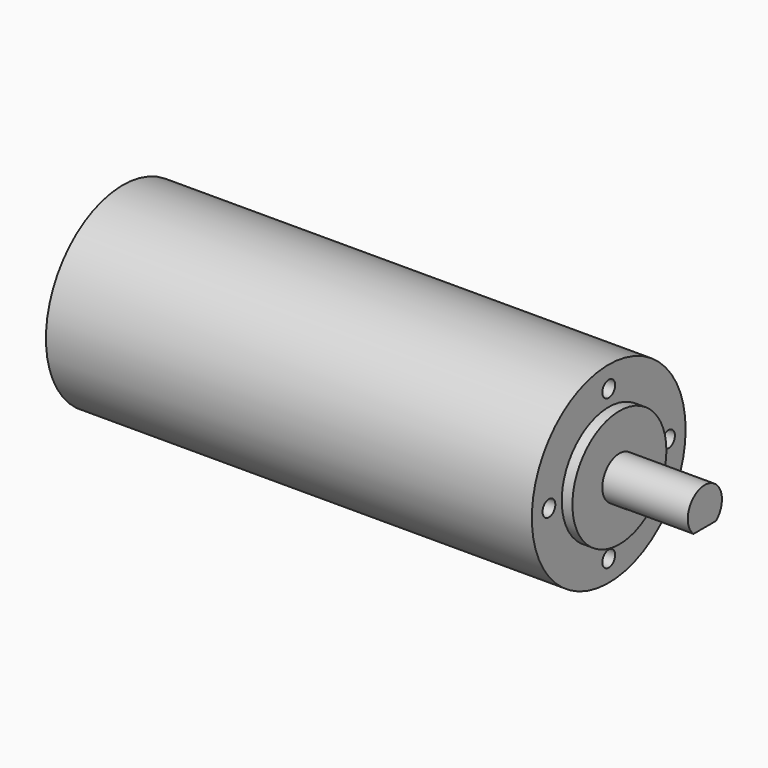
from build123d import *

# Parameters (mm, degrees)
F0_R            = 18
F1_DEPTH        = 91
F2_R            = 11
F3_DEPTH        = 2
F4_R            = 4
F5_DEPTH        = 18
F6_R            = 1.5
F7_DEPTH        = 5
F7_COPIES_COUNT = 4
F9_START        = 5
F8_W            = 20
F8_H            = 10
F9_DEPTH        = 20


# Not quite as in the source:
# - a pattern or mirror of a feature is missing from the dataset's text; its kind, count and spacing are read off the source's solid


with BuildPart() as f1:
    # F0 (on Right) → F1 (new body)
    with BuildSketch(Plane.YZ):
        Circle(F0_R)
    extrude(amount=-F1_DEPTH)

    # F2 (on Right) → F3 (join)
    with BuildSketch(Plane.YZ):
        Circle(F2_R)
    extrude(amount=F3_DEPTH)

    # F4 (on Right) → F5 (join)
    with BuildSketch(Plane.YZ):
        Circle(F4_R)
    extrude(amount=F5_DEPTH)

    # F6 (on Right) → F7 (cut)
    with BuildSketch(Plane.YZ):
        with Locations((14, 0)):
            Circle(F6_R)
    f7 = extrude(amount=-F7_DEPTH, mode=Mode.SUBTRACT)

    # F7_copies: F7 ×4 about axis
    f7_copies_axis = Axis((0, 0, 0), (1, 0, 0))
    for i in range(1, F7_COPIES_COUNT):
        add(f7.rotate(f7_copies_axis, i * 360 / F7_COPIES_COUNT), mode=Mode.SUBTRACT)

    # F8 (on Right) → F9 (cut)
    with BuildSketch(Plane.YZ.offset(F9_START)):
        with Locations((0, -8)):
            Rectangle(F8_W, F8_H)
    extrude(amount=F9_DEPTH, mode=Mode.SUBTRACT)


solid = f1.part
